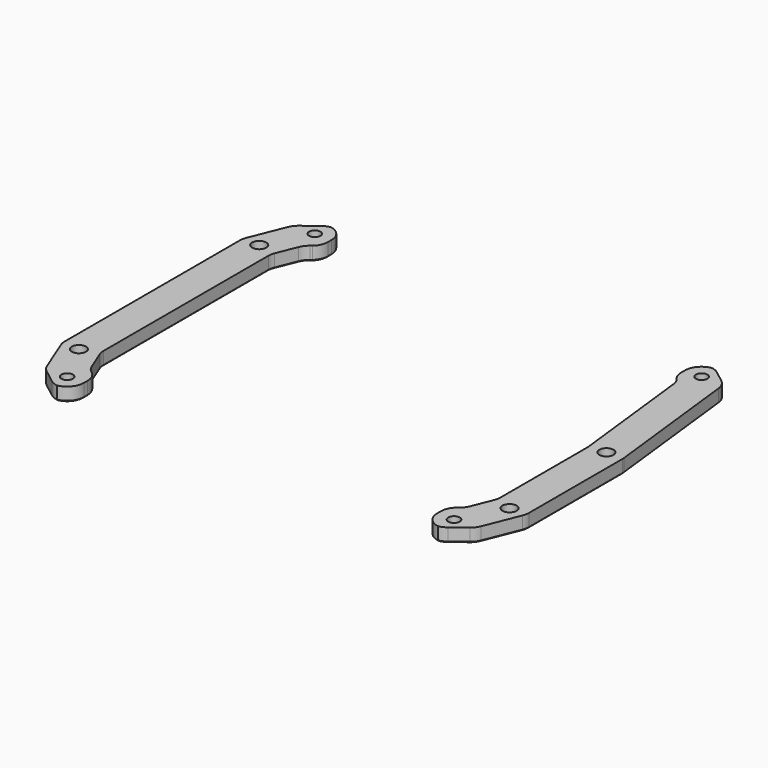
from build123d import *

# Parameters (mm, degrees)
F3_DEPTH        = 4
F0_R            = 2.1
F4_DEPTH        = 4.001
F5_R            = 1.7
F6_DEPTH        = 4.001
F7_W            = 105
F7_H            = 4
F8_DEPTH        = 102.001
F9_T1_DEPTH     = 29
F9_T3_DEPTH     = 12.5030486671
F9_T5_DEPTH     = 10.8462610372
F9_T7_DEPTH     = 8.8145600892
F9_T9_DEPTH     = 22.3246460663
F9_T11_DEPTH    = 4
F9_S1_T1_DEPTH  = 4
F9_S1_T3_DEPTH  = 12.5030486671
F9_S1_T5_DEPTH  = 10.8462610372
F9_S1_T7_DEPTH  = 8.8145600892
F9_S1_T9_DEPTH  = 29
F9_S1_T11_DEPTH = 22.3246460663
F9_S1_T13_DEPTH = 14.5795623731
F9_S1_T15_DEPTH = 5.4320670893
F10_C1_SIZE     = 0.3
F10_C2_SIZE     = 0.3
F10_C3_SIZE     = 0.2999
F10_C4_SIZE     = 0.3
F10_C5_SIZE     = 0.3
F10_C6_SIZE     = 0.3
F10_C7_SIZE     = 0.3
F10_S1_C1_SIZE  = 0.3
F10_S1_C2_SIZE  = 0.3
F10_S1_C3_SIZE  = 0.3
F10_S1_C4_SIZE  = 0.3
F10_S1_C5_SIZE  = 0.3
F10_S1_C6_SIZE  = 0.3


# Not quite as in the source:
# - a fillet or chamfer that OpenCascade refuses, or shapes differently, is made with other operations: its cross-section is extruded or revolved along the edge and cut away or added
# - a fillet or chamfer is up to 0.001 mm smaller than in the source, because OpenCascade refuses the exact size


with BuildPart() as f3:
    # F2 (on Top) → F3 (new body)
    with BuildSketch(Plane.XY):
        Polygon((-64, 46), (-69, 33.5), (-69, -33.5), (-64, -46), (-57.5, -51), (57.5, -51), (64, -46), (69, -33.5), (69, 2.5), (64, 46), (57.5, 51), (-57.5, 51), align=None)
        Polygon((59, -31.5741759643), (55.732288098, -39.7434557193), (54.0987805331, -41), (-54.0987805331, -41), (-55.732288098, -39.7434557193), (-59, -31.5741759643), (-59, 31.5741759643), (-55.732288098, 39.7434557193), (-54.0987805331, 41), (54.0987805331, 41), (54.5486464191, 40.6539493185), (59, 1.9271731643), align=None, mode=Mode.SUBTRACT)
    extrude(amount=F3_DEPTH)

    # F0 (on Top) → F4 (cut, through all)
    with BuildSketch(Plane.XY):
        with Locations((-64, 33.5)):
            Circle(F0_R)
        with Locations((-64, -33.5)):
            Circle(F0_R)
        with Locations((64, -33.5)):
            Circle(F0_R)
        with Locations((64, 2.5)):
            Circle(F0_R)
    extrude(amount=F4_DEPTH, mode=Mode.SUBTRACT)

    # F5 (on face) → F6 (cut, through all)
    with BuildSketch(Plane.XY.offset(4)):
        with Locations((-57.5, 46)):
            Circle(F5_R)
        with Locations((57.5, 46)):
            Circle(F5_R)
        with Locations((57.5, -46)):
            Circle(F5_R)
        with Locations((-57.5, -46)):
            Circle(F5_R)
    extrude(amount=-F6_DEPTH, mode=Mode.SUBTRACT)

    # F7 (on face) → F8 (cut, through all)
    with BuildSketch(Plane.XZ.offset(51)):
        with Locations((0, 2)):
            Rectangle(F7_W, F7_H)
    extrude(amount=-F8_DEPTH, mode=Mode.SUBTRACT)

    # F9: fillet of radius 5 on 14 edges, made by hand

    # F9_s2 → F9_t1 (cut)
    with BuildSketch(Plane.XY.offset(-12.5)):
        with BuildLine():
            ThreePointArc((-52.5, -46), (-53.9644660941, -49.5355339059), (-57.5, -51))
            Line((-57.5, -51), (-57.5, -51.1))
            Line((-57.5, -51.1), (-52.4, -51.1))
            Line((-52.4, -51.1), (-52.4, -46))
            Line((-52.4, -46), (-52.5, -46))
        make_face()
        with BuildLine():
            ThreePointArc((-57.5, 51), (-53.9644660941, 49.5355339059), (-52.5, 46))
            Line((-52.5, 46), (-52.4, 46))
            Line((-52.4, 46), (-52.4, 51.1))
            Line((-52.4, 51.1), (-57.5, 51.1))
            Line((-57.5, 51.1), (-57.5, 51))
        make_face()
    extrude(amount=F9_T1_DEPTH, mode=Mode.SUBTRACT)

    # F9_s4 → F9_t3 (cut)
    with BuildSketch(Plane.XY.offset(-4.2515243336)):
        with BuildLine():
            ThreePointArc((-55.7993902666, -51), (-57.4094213645, -50.7336877658), (-58.8479440708, -49.9631199455))
            Line((-58.8479440708, -49.9631199455), (-58.9089151469, -50.0423823444))
            Line((-58.9089151469, -50.0423823444), (-57.5340121947, -51.1))
            Line((-57.5340121947, -51.1), (-55.7993902666, -51.1))
            Line((-55.7993902666, -51.1), (-55.7993902666, -51))
        make_face()
        with BuildLine():
            ThreePointArc((-58.8479440708, 49.9631199455), (-57.4094213645, 50.7336877658), (-55.7993902666, 51))
            Line((-55.7993902666, 51), (-55.7993902666, 51.1))
            Line((-55.7993902666, 51.1), (-57.5340121947, 51.1))
            Line((-57.5340121947, 51.1), (-58.9089151469, 50.0423823444))
            Line((-58.9089151469, 50.0423823444), (-58.8479440708, 49.9631199455))
        make_face()
    extrude(amount=F9_T3_DEPTH, mode=Mode.SUBTRACT)

    # F9_s6 → F9_t5 (cut)
    with BuildSketch(Plane.XY.offset(-3.4231305186)):
        with BuildLine():
            ThreePointArc((-64.5085275034, -44.7286812414), (-63.8531997769, -45.8889097604), (-62.9146978532, -46.8348478052))
            Line((-62.9146978532, -46.8348478052), (-62.9756689293, -46.9141102041))
            Line((-62.9756689293, -46.9141102041), (-64.082677119, -46.0625654428))
            Line((-64.082677119, -46.0625654428), (-64.6013751725, -44.7658203091))
            Line((-64.6013751725, -44.7658203091), (-64.5085275034, -44.7286812414))
        make_face()
        with BuildLine():
            ThreePointArc((-64.5085275034, 44.7286812414), (-63.8531997769, 45.8889097604), (-62.9146978532, 46.8348478052))
            Line((-62.9146978532, 46.8348478052), (-62.9756689293, 46.9141102041))
            Line((-62.9756689293, 46.9141102041), (-64.082677119, 46.0625654428))
            Line((-64.082677119, 46.0625654428), (-64.6013751725, 44.7658203091))
            Line((-64.6013751725, 44.7658203091), (-64.5085275034, 44.7286812414))
        make_face()
    extrude(amount=F9_T5_DEPTH, mode=Mode.SUBTRACT)

    # F9_s8 → F9_t7 (cut)
    with BuildSketch(Plane.XY.offset(-2.4072800446)):
        with BuildLine():
            ThreePointArc((-69, -32.5370879822), (-68.9097819337, -33.4826255879), (-68.6423834544, -34.3940413639))
            Line((-68.6423834544, -34.3940413639), (-68.7352311235, -34.4311804316))
            Line((-68.7352311235, -34.4311804316), (-69.1, -33.5192582404))
            Line((-69.1, -33.5192582404), (-69.1, -32.5370879822))
            Line((-69.1, -32.5370879822), (-69, -32.5370879822))
        make_face()
        with BuildLine():
            ThreePointArc((-68.6423834544, 34.3940413639), (-68.9097819337, 33.4826255879), (-69, 32.5370879822))
            Line((-69, 32.5370879822), (-69.1, 32.5370879822))
            Line((-69.1, 32.5370879822), (-69.1, 33.5192582404))
            Line((-69.1, 33.5192582404), (-68.7352311235, 34.4311804316))
            Line((-68.7352311235, 34.4311804316), (-68.6423834544, 34.3940413639))
        make_face()
    extrude(amount=F9_T7_DEPTH, mode=Mode.SUBTRACT)

    # F9_s10 → F9_t9 (cut)
    with BuildSketch(Plane.XY.offset(-9.1623230332)):
        with BuildLine():
            ThreePointArc((-54.0987805331, -41), (-52.9170916803, -42.6656915253), (-52.5, -44.6649292133))
            Line((-52.5, -44.6649292133), (-52.4, -44.6649292133))
            Line((-52.4, -44.6649292133), (-52.4, -41))
            Line((-52.4, -41), (-52.5, -40.9))
            ThreePointArc((-52.5, -40.9), (-53.2993902666, -40.9), (-54.0307561438, -40.9267014157))
            Line((-54.0307561438, -40.9267014157), (-54.0987805331, -41))
        make_face()
        with BuildLine():
            ThreePointArc((-52.5, 44.6649292133), (-52.9170916803, 42.6656915253), (-54.0987805331, 41))
            Line((-54.0987805331, 41), (-54.0307561438, 40.9267014157))
            ThreePointArc((-54.0307561438, 40.9267014157), (-53.2993902666, 40.9), (-52.5, 40.9))
            Line((-52.5, 40.9), (-52.4, 41))
            Line((-52.4, 41), (-52.4, 44.6649292133))
            Line((-52.4, 44.6649292133), (-52.5, 44.6649292133))
        make_face()
    extrude(amount=F9_T9_DEPTH, mode=Mode.SUBTRACT)

    # F9_s12 → F9_t11 (join)
    with BuildSketch(Plane.XY):
        with BuildLine():
            ThreePointArc((-56.2408156014, -38.4721369608), (-55.5854878749, -39.6323654798), (-54.6469859512, -40.5783035245))
            Line((-54.6469859512, -40.5783035245), (-54.7079570273, -40.6575659235))
            Line((-54.7079570273, -40.6575659235), (-55.814965217, -39.8060211622))
            Line((-55.814965217, -39.8060211622), (-56.3336632705, -38.5092760284))
            Line((-56.3336632705, -38.5092760284), (-56.2408156014, -38.4721369608))
        make_face()
        with BuildLine():
            ThreePointArc((-59, -30.6112639465), (-58.9097819337, -31.5568015523), (-58.6423834544, -32.4682173283))
            Line((-58.6423834544, -32.4682173283), (-58.7352311235, -32.5053563959))
            Line((-58.7352311235, -32.5053563959), (-59.1, -31.5934342047))
            Line((-59.1, -31.5934342047), (-59.1, -30.6112639465))
            Line((-59.1, -30.6112639465), (-59, -30.6112639465))
        make_face()
        with BuildLine():
            ThreePointArc((-58.6423834544, 32.4682173283), (-58.9097819337, 31.5568015523), (-59, 30.6112639465))
            Line((-59, 30.6112639465), (-59.1, 30.6112639465))
            Line((-59.1, 30.6112639465), (-59.1, 31.5934342047))
            Line((-59.1, 31.5934342047), (-58.7352311235, 32.5053563959))
            Line((-58.7352311235, 32.5053563959), (-58.6423834544, 32.4682173283))
        make_face()
        with BuildLine():
            ThreePointArc((-54.6469859512, 40.5783035245), (-55.5854878749, 39.6323654798), (-56.2408156014, 38.4721369608))
            Line((-56.2408156014, 38.4721369608), (-56.3336632705, 38.5092760284))
            Line((-56.3336632705, 38.5092760284), (-55.814965217, 39.8060211622))
            Line((-55.814965217, 39.8060211622), (-54.7079570273, 40.6575659235))
            Line((-54.7079570273, 40.6575659235), (-54.6469859512, 40.5783035245))
        make_face()
    extrude(amount=F9_T11_DEPTH)

    # F9#s1: fillet of radius 5 on 14 edges, made by hand

    # F9_s1_s2 → F9_s1_t1 (join)
    with BuildSketch(Plane.XY):
        with BuildLine():
            ThreePointArc((54.6469859512, -40.5783035245), (55.5854878749, -39.6323654798), (56.2408156014, -38.4721369608))
            Line((56.2408156014, -38.4721369608), (55.732288098, -39.7434557193))
            Line((55.732288098, -39.7434557193), (54.6469859512, -40.5783035245))
        make_face()
        with BuildLine():
            ThreePointArc((58.6423834544, -32.4682173283), (58.9097819337, -31.5568015523), (59, -30.6112639465))
            Line((59, -30.6112639465), (59, -31.5741759643))
            Line((59, -31.5741759643), (58.6423834544, -32.4682173283))
        make_face()
        with BuildLine():
            ThreePointArc((59, 1.6407597464), (58.9918168684, 1.9267044125), (58.9672942592, 2.2117131095))
            Line((58.9672942592, 2.2117131095), (59, 1.9271731643))
            Line((59, 1.9271731643), (59, 1.6407597464))
        make_face()
        with BuildLine():
            ThreePointArc((54.7292655037, 39.0825632824), (54.511784567, 40.0734272586), (54.0987805331, 41))
            Line((54.0987805331, 41), (54.5486464191, 40.6539493185))
            Line((54.5486464191, 40.6539493185), (54.7292655037, 39.0825632824))
        make_face()
    extrude(amount=F9_S1_T1_DEPTH)

    # F9_s1_s4 → F9_s1_t3 (cut)
    with BuildSketch(Plane.XY.offset(-4.2515243336)):
        with BuildLine():
            ThreePointArc((58.8479440708, -49.9631199455), (57.4094213645, -50.7336877658), (55.7993902666, -51))
            Line((55.7993902666, -51), (57.5, -51))
            Line((57.5, -51), (58.8479440708, -49.9631199455))
        make_face()
        with BuildLine():
            ThreePointArc((55.7993902666, 51), (57.4094213645, 50.7336877658), (58.8479440708, 49.9631199455))
            Line((58.8479440708, 49.9631199455), (57.5, 51))
            Line((57.5, 51), (55.7993902666, 51))
        make_face()
    extrude(amount=F9_S1_T3_DEPTH, mode=Mode.SUBTRACT)

    # F9_s1_s6 → F9_s1_t5 (cut)
    with BuildSketch(Plane.XY.offset(-3.4231305186)):
        with BuildLine():
            ThreePointArc((64.5085275034, -44.7286812414), (63.8531997769, -45.8889097604), (62.9146978532, -46.8348478052))
            Line((62.9146978532, -46.8348478052), (64, -46))
            Line((64, -46), (64.5085275034, -44.7286812414))
        make_face()
    extrude(amount=F9_S1_T5_DEPTH, mode=Mode.SUBTRACT)

    # F9_s1_s8 → F9_s1_t7 (cut)
    with BuildSketch(Plane.XY.offset(-2.4072800446)):
        with BuildLine():
            ThreePointArc((69, -32.5370879822), (68.9097819337, -33.4826255879), (68.6423834544, -34.3940413639))
            Line((68.6423834544, -34.3940413639), (69, -33.5))
            Line((69, -33.5), (69, -32.5370879822))
        make_face()
    extrude(amount=F9_S1_T7_DEPTH, mode=Mode.SUBTRACT)

    # F9_s1_s10 → F9_s1_t9 (cut)
    with BuildSketch(Plane.XY.offset(-12.5)):
        with BuildLine():
            ThreePointArc((57.5, -51), (53.9644660941, -49.5355339059), (52.5, -46))
            Line((52.5, -46), (52.5, -51))
            Line((52.5, -51), (57.5, -51))
        make_face()
        with BuildLine():
            ThreePointArc((57.5, 51), (53.9644660941, 49.5355339059), (52.5, 46))
            Line((52.5, 46), (52.5, 51))
            Line((52.5, 51), (57.5, 51))
        make_face()
    extrude(amount=F9_S1_T9_DEPTH, mode=Mode.SUBTRACT)

    # F9_s1_s12 → F9_s1_t11 (cut)
    with BuildSketch(Plane.XY.offset(-9.1623230332)):
        with BuildLine():
            ThreePointArc((52.5, -44.6649292133), (52.9170916803, -42.6656915253), (54.0987805331, -41))
            Line((54.0987805331, -41), (52.5, -41))
            Line((52.5, -41), (52.5, -44.6649292133))
        make_face()
        with BuildLine():
            ThreePointArc((54.0987805331, 41), (52.9170916803, 42.6656915253), (52.5, 44.6649292133))
            Line((52.5, 44.6649292133), (52.5, 41))
            Line((52.5, 41), (54.0987805331, 41))
        make_face()
    extrude(amount=F9_S1_T11_DEPTH, mode=Mode.SUBTRACT)

    # F9_s1_s14 → F9_s1_t13 (cut)
    with BuildSketch(Plane.XY.offset(-5.2897811865)):
        with BuildLine():
            ThreePointArc((62.3228770138, 47.2900946048), (63.626351883, 45.7886501914), (64.2416174687, 43.8979280224))
            Line((64.2416174687, 43.8979280224), (64, 46))
            Line((64, 46), (62.3228770138, 47.2900946048))
        make_face()
    extrude(amount=F9_S1_T13_DEPTH, mode=Mode.SUBTRACT)

    # F9_s1_s16 → F9_s1_t15 (cut)
    with BuildSketch(Plane.XY.offset(-0.7160335447)):
        with BuildLine():
            ThreePointArc((68.9672942592, 2.7845399453), (68.9918168684, 2.4995312483), (69, 2.2135865821))
            Line((69, 2.2135865821), (69, 2.5))
            Line((69, 2.5), (68.9672942592, 2.7845399453))
        make_face()
    extrude(amount=F9_S1_T15_DEPTH, mode=Mode.SUBTRACT)

    # F10: chamfer of 0.3 on 29 edges, made by hand

    # F10_c1
    f10_c1_edges = [f3.edges().sort_by_distance(p)[0] for p in [
        (57.8075291455, 50.5790149861, 0),
        (60.5854105423, 48.6266072752, 0),
        (63.626351883, 45.7886501914, 0),
        (66.6044558639, 23.3412339838, 0),
        (68.9918168684, 2.4995312483, 0),
        (69, -15.1617507, 0),
        (68.9097819337, -33.482625588, 0),
        (66.5754554789, -39.5613613027, 0),
        (63.8531997769, -45.8889097604, 0),
        (60.881320962, -48.3989838754, 0),
        (57.8075291455, -50.5790149861, 0),
    ]]
    chamfer(f10_c1_edges, length=F10_C1_SIZE)

    # F10_c2
    f10_c2_edges = [f3.edges().sort_by_distance(p)[0] for p in [
        (53.4055280093, -48.869721087, 0),
        (52.5, -45.3324646066, 0),
        (52.9170916803, -42.6656915254, 0),
    ]]
    chamfer(f10_c2_edges, length=F10_C2_SIZE)

    # F10_c3 (size 0.3 in the source; OpenCascade refuses exactly that, so slightly less here)
    f10_c3_edges = [f3.edges().sort_by_distance(p)[0] for p in [
        (52.9170916803, 42.6656915254, 0),
        (52.5, 45.3324646067, 0),
        (53.4055280093, 48.869721087, 0),
    ]]
    chamfer(f10_c3_edges, length=F10_C3_SIZE)

    # F10_c4
    f10_c4_edges = [f3.edges().sort_by_distance(p)[0] for p in [
        (55.8, -46, 0),
    ]]
    chamfer(f10_c4_edges, length=F10_C4_SIZE)

    # F10_c5
    f10_c5_edges = [f3.edges().sort_by_distance(p)[0] for p in [
        (61.9, -33.5, 0),
    ]]
    chamfer(f10_c5_edges, length=F10_C5_SIZE)

    # F10_c6
    f10_c6_edges = [f3.edges().sort_by_distance(p)[0] for p in [
        (55.8, 46, 0),
    ]]
    chamfer(f10_c6_edges, length=F10_C6_SIZE)

    # F10_c7
    f10_c7_edges = [f3.edges().sort_by_distance(p)[0] for p in [
        (61.9, 2.5, 0),
    ]]
    chamfer(f10_c7_edges, length=F10_C7_SIZE)

    # F10#s1: chamfer of 0.3 on 30 edges, made by hand

    # F10_s1_c1
    f10_s1_c1_edges = [f3.edges().sort_by_distance(p)[0] for p in [
        (-66.5754554789, 39.5613613027, 0),
        (-57.8075291455, 50.5790149861, 0),
        (-60.881320962, 48.3989838754, 0),
        (-63.8531997769, 45.8889097604, 0),
        (-68.9097819337, 33.482625588, 0),
        (-69, 0, 0),
        (-68.9097819337, -33.482625588, 0),
        (-66.5754554789, -39.5613613027, 0),
        (-63.8531997769, -45.8889097604, 0),
        (-60.881320962, -48.3989838754, 0),
        (-57.8075291455, -50.5790149861, 0),
    ]]
    chamfer(f10_s1_c1_edges, length=F10_S1_C1_SIZE)

    # F10_s1_c2
    f10_s1_c2_edges = [f3.edges().sort_by_distance(p)[0] for p in [
        (-53.4055280093, 48.869721087, 0),
        (-52.9170916803, 42.6656915254, 0),
        (-52.5, 45.3324646066, 0),
    ]]
    chamfer(f10_s1_c2_edges, length=F10_S1_C2_SIZE)

    # F10_s1_c3
    f10_s1_c3_edges = [f3.edges().sort_by_distance(p)[0] for p in [
        (-66.1, -33.5, 0),
    ]]
    chamfer(f10_s1_c3_edges, length=F10_S1_C3_SIZE)

    # F10_s1_c4
    f10_s1_c4_edges = [f3.edges().sort_by_distance(p)[0] for p in [
        (-59.2, -46, 0),
    ]]
    chamfer(f10_s1_c4_edges, length=F10_S1_C4_SIZE)

    # F10_s1_c5
    f10_s1_c5_edges = [f3.edges().sort_by_distance(p)[0] for p in [
        (-66.1, 33.5, 0),
    ]]
    chamfer(f10_s1_c5_edges, length=F10_S1_C5_SIZE)

    # F10_s1_c6
    f10_s1_c6_edges = [f3.edges().sort_by_distance(p)[0] for p in [
        (-59.2, 46, 0),
    ]]
    chamfer(f10_s1_c6_edges, length=F10_S1_C6_SIZE)


solid = f3.part
